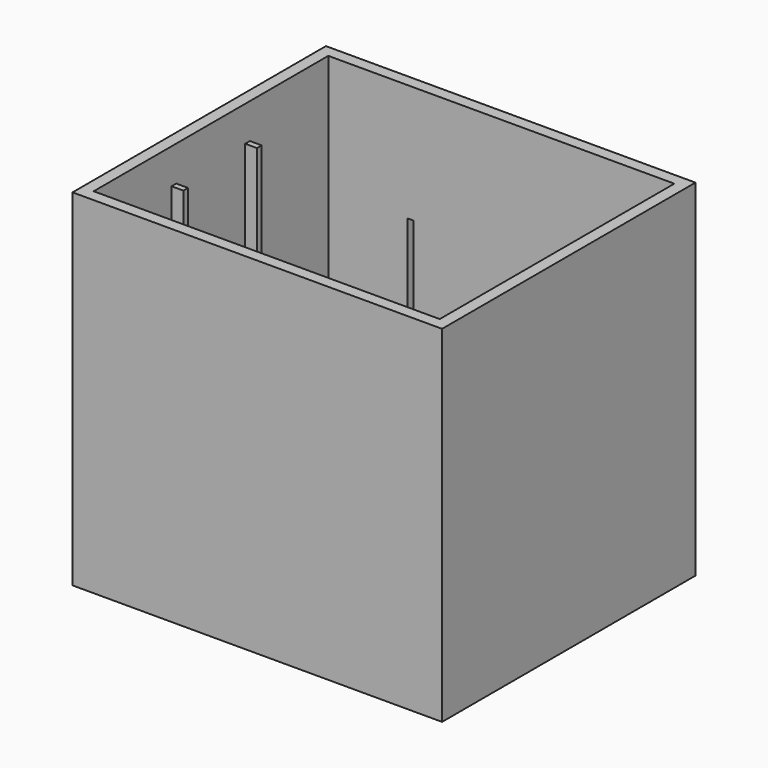
from build123d import *

# Parameters (mm, degrees)
F0_W     = 63
F0_H     = 54
F0_W_2   = 59
F0_H_2   = 50
F1_DEPTH = 59
F2_DEPTH = 2
F3_W     = 1
F3_H     = 51
F4_DEPTH = 2
F5_START = 57
F5_DEPTH = 2
F6_W     = 1
F6_H     = 19
F7_DEPTH = 3


with BuildPart() as f1:
    # F0 (on Top) → F1 (new body)
    with BuildSketch(Plane.XY):
        with Locations((-808.1280109427, -717.9987351179)):
            Rectangle(F0_W, F0_H)
        with Locations((-808.1280109427, -717.9987351179)):
            Rectangle(F0_W_2, F0_H_2, mode=Mode.SUBTRACT)
    extrude(amount=F1_DEPTH)

    # F0 (on Top) → F2 (join)
    with BuildSketch(Plane.XY):
        with Locations((-808.1280109427, -717.9987351179)):
            Rectangle(F0_W_2, F0_H_2)
    extrude(amount=F2_DEPTH)

    # F3 (on face) → F4 (join)
    with BuildSketch(Plane.YZ.offset(-837.6280109427)):
        with Locations((-710.1987351179, 27.5)):
            Rectangle(F3_W, F3_H)
        with Locations((-725.8987351179, 27.5)):
            Rectangle(F3_W, F3_H)
    extrude(amount=F4_DEPTH)

    # F3 (on face) → F5 (join)
    with BuildSketch(Plane.YZ.offset(-837.6280109427).offset(F5_START)):
        with Locations((-710.1987351179, 27.5)):
            Rectangle(F3_W, F3_H)
        with Locations((-725.8987351179, 27.5)):
            Rectangle(F3_W, F3_H)
    extrude(amount=F5_DEPTH)

    # F6 (on face) → F7 (cut)
    with BuildSketch(Plane(origin=(0, -690.9987351179, 0), x_dir=(-1, 0, 0), z_dir=(0, 1, 0))):
        with Locations((823.6280109427, 29.5)):
            Rectangle(F6_W, F6_H)
        with Locations((792.6280109427, 29.5)):
            Rectangle(F6_W, F6_H)
    extrude(amount=-F7_DEPTH, mode=Mode.SUBTRACT)


solid = f1.part
